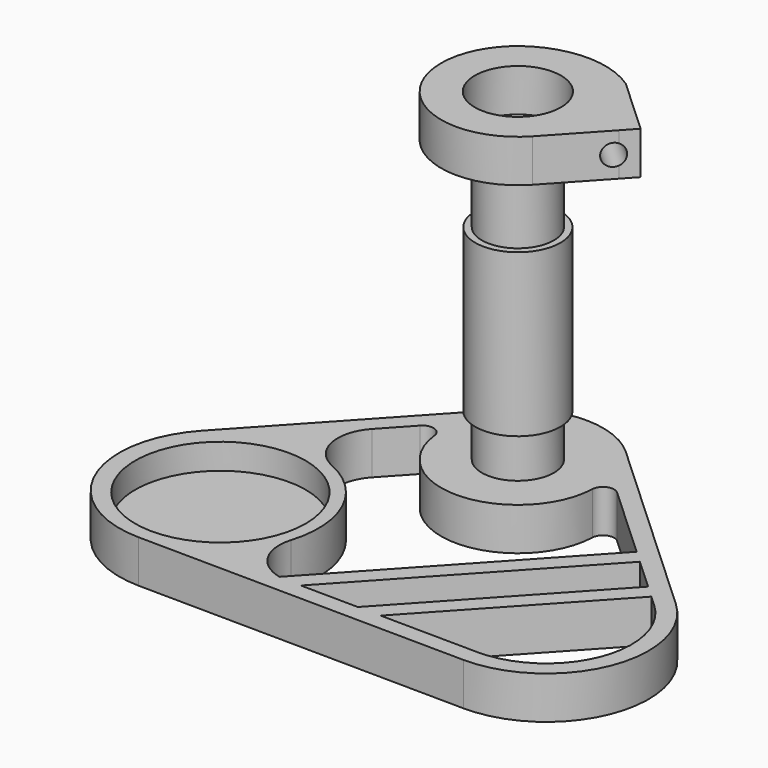
from build123d import *

# Parameters (mm, degrees)
F0_R     = 10
F0_R_2   = 5
F0_R_3   = 4.225
F1_DEPTH = 5
F2_DEPTH = 33
F3_DEPTH = 24
F4_DEPTH = 3
F5_DEPTH = 5
F6_R     = 5.05
F7_DEPTH = 5
F8_R     = 1.25
F9_DEPTH = 37.3461542928


# Not quite as in the source:
# - a feature names something its author has since deleted; it is built from what else it names


with BuildPart() as f1:
    # F0 (on Top) → F1 (new body)
    with BuildSketch(Plane.XY):
        with BuildLine():
            ThreePointArc((37.8886156331, -47.7045562268), (30.7058016888, -45.0614846038), (23.757851373, -48.271567184))
            Line((23.757851373, -48.271567184), (4.9458403192, -68.6563901516))
            ThreePointArc((4.9458403192, -68.6563901516), (2.7469798041, -81.5500736227), (13.6377095304, -88.793972231))
            Line((13.6377095304, -88.793972231), (52.0294167207, -89.1996541952))
            ThreePointArc((52.0294167207, -89.1996541952), (63.3093775894, -81.6282933397), (60.2944646217, -68.3816589671))
            Line((60.2944646217, -68.3816589671), (37.8886156331, -47.7045562268))
        make_face()
        with Locations((13.8766520367, -77.1243319886)):
            Circle(F0_R, mode=Mode.SUBTRACT)
        with BuildLine():
            ThreePointArc((19.9178327929, -55.3816736395), (21.2773906019, -55.0259616092), (22.1692135687, -56.1120464494))
            ThreePointArc((22.1692135687, -56.1120464494), (31.4675825452, -64.046207144), (40.1003485207, -55.3925418418))
            ThreePointArc((40.1003485207, -55.3925418418), (40.9022839083, -54.2384932646), (42.285971428, -54.4841298503))
            Line((42.285971428, -54.4841298503), (51.0236458615, -62.5476400554))
            Line((51.0236458615, -62.5476400554), (52.4934233832, -63.9040153856))
            Line((52.4934233832, -63.9040153856), (56.1678671876, -67.2949537114))
            Line((56.1678671876, -67.2949537114), (57.6376447093, -68.6513290416))
            Line((57.6376447093, -68.6513290416), (58.9380892914, -69.8514364888))
            ThreePointArc((58.9380892914, -69.8514364888), (58.9480578825, -69.8606484779), (58.9580139608, -69.8698739891))
            ThreePointArc((58.9580139608, -69.8698739891), (61.4454997037, -80.9029104703), (52.0505493739, -87.1997658456))
            Line((52.0505493739, -87.1997658456), (40.6316839441, -87.0791036481))
            Line((40.6316839441, -87.0791036481), (37.9364663461, -87.0506235088))
            Line((37.9364663461, -87.0506235088), (31.1984223512, -86.9794231605))
            Line((31.1984223512, -86.9794231605), (29.5984604838, -86.962516497))
            ThreePointArc((29.5984604838, -86.962516497), (29.0944782553, -86.9316947288), (28.5961743715, -86.8502005114))
            ThreePointArc((28.5961743715, -86.8502005114), (25.3379647523, -84.491670283), (24.8710981532, -80.4965945217))
            ThreePointArc((24.8710981532, -80.4965945217), (24.3410382572, -72.3549902073), (18.5438366298, -66.6139852782))
            ThreePointArc((18.5438366298, -66.6139852782), (15.67652582, -63.0562363009), (16.8986035181, -58.6533309914))
            Line((16.8986035181, -58.6533309914), (19.9178327929, -55.3816736395))
        make_face(mode=Mode.SUBTRACT)
        with Locations((31.1067389816, -55.0534438355)):
            Circle(F0_R_2, mode=Mode.SUBTRACT)
        with Locations((13.8766520367, -77.1243319886)):
            Circle(F0_R)
        with Locations((31.1067389816, -55.0534438355)):
            Circle(F0_R_2)
        with Locations((31.1067389816, -55.0534438355)):
            Circle(F0_R_3, mode=Mode.SUBTRACT)
        with BuildLine():
            Line((52.4934233832, -63.9040153856), (51.0236458615, -62.5476400554))
            Line((51.0236458615, -62.5476400554), (28.5961743715, -86.8502005114))
            ThreePointArc((28.5961743715, -86.8502005114), (29.0944782553, -86.9316947288), (29.5984604838, -86.962516497))
            Line((29.5984604838, -86.962516497), (31.1984223512, -86.9794231605))
            Line((31.1984223512, -86.9794231605), (52.4934233832, -63.9040153856))
        make_face()
        Polygon((57.6376447093, -68.6513290416), (56.1678671876, -67.2949537114), (37.9364663461, -87.0506235088), (40.6316839441, -87.0791036481), align=None)
    extrude(amount=-F1_DEPTH)



with BuildPart() as f2:
    # F0 (on Top) → F2 (new body)
    with BuildSketch(Plane.XY):
        with Locations((31.1067389816, -55.0534438355)):
            Circle(F0_R_3)
    extrude(amount=F2_DEPTH)


with BuildPart() as f1_1:
    add(f1.part)

    add(f2.part)  # F3 merges F2
    # F0 (on Top) → F3 (join)
    with BuildSketch(Plane.XY):
        with Locations((31.1067389816, -55.0534438355)):
            Circle(F0_R_2)
        with Locations((31.1067389816, -55.0534438355)):
            Circle(F0_R_3, mode=Mode.SUBTRACT)
    extrude(amount=F3_DEPTH)

    # F0 (on Top) → F4 (cut)
    with BuildSketch(Plane.XY):
        with Locations((13.8766520367, -77.1243319886)):
            Circle(F0_R)
    extrude(amount=-F4_DEPTH, mode=Mode.SUBTRACT)

    # F0 (on Top) → F5 (cut)
    with BuildSketch(Plane.XY):
        with Locations((31.1067389816, -55.0534438355)):
            Circle(F0_R_2)
        with Locations((31.1067389816, -55.0534438355)):
            Circle(F0_R_3, mode=Mode.SUBTRACT)
    extrude(amount=F5_DEPTH, mode=Mode.SUBTRACT)


with BuildPart() as f7:
    # F6 (on face) → F7 (new body)
    with BuildSketch(Plane.XY.offset(33)):
        with BuildLine():
            ThreePointArc((26.5920293669, -47.2677263287), (23.0571330032, -51.0280440303), (22.1692135687, -56.1120464494))
            ThreePointArc((22.1692135687, -56.1120464494), (28.3295249008, -63.6142312963), (37.7207378294, -61.1571328217))
            Line((37.7207378294, -61.1571328217), (43.1462391506, -55.2780227348))
            Line((43.1462391506, -55.2780227348), (44.5026144809, -53.8082452131))
            Line((44.5026144809, -53.8082452131), (37.8886156331, -47.7045562268))
            ThreePointArc((37.8886156331, -47.7045562268), (32.303661001, -45.8481837024), (26.5920293669, -47.2677263287))
        make_face()
        with Locations((31.1067389816, -55.0534438355)):
            Circle(F6_R, mode=Mode.SUBTRACT)
    extrude(amount=F7_DEPTH)

    # F8 (on face) → F9 (cut, through all)
    with BuildSketch(Plane(origin=(50.851773792, -46.9282530538, 0), x_dir=(0.6781876651, 0.7348887609, 0), z_dir=(0.7348887609, -0.6781876651, 0))):
        with Locations((-11.8619504415, 35.5)):
            Circle(F8_R)
    extrude(amount=-F9_DEPTH, mode=Mode.SUBTRACT)


solid = Compound([f1_1.part, f7.part])
